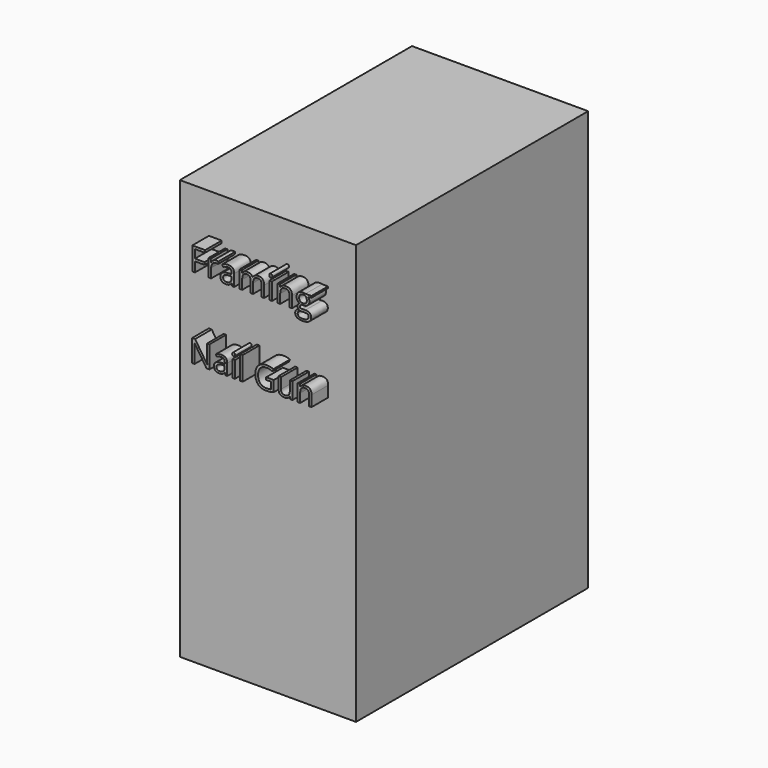
from build123d import *

# Parameters (mm, degrees)
F0_W           = 215.9
F0_H           = 514.35
F1_DEPTH       = 355.6
F2_TEXT_SIZE   = 37.9517509728
F2_TEXT_SIZE_2 = 39.4196338358
F3_DEPTH       = 25.4


# Not quite as in the source:
# - Text() gives the source's letters only with a copy of the font that has no kerning and outlines rounded to 1/6400 em; it was checked with that copy


with BuildPart() as f1:
    # F0 (on Front) → F1 (new body)
    with BuildSketch(Plane.XZ):
        Rectangle(F0_W, F0_H)
    extrude(amount=F1_DEPTH)

    # F2 (on face) → F3 (join)
    with BuildSketch(Plane.XZ.offset(355.6)):
        with Locations((-76.2, 81.6031581267)):
            Text('Nail Gun', F2_TEXT_SIZE, font='Open Sans', text_align=(TextAlign.LEFT, TextAlign.BOTTOM))
        with Locations((-76.2, 180.4647903273)):
            Text('Framing', F2_TEXT_SIZE_2, font='Open Sans', text_align=(TextAlign.LEFT, TextAlign.BOTTOM))
    extrude(amount=F3_DEPTH)


solid = f1.part
